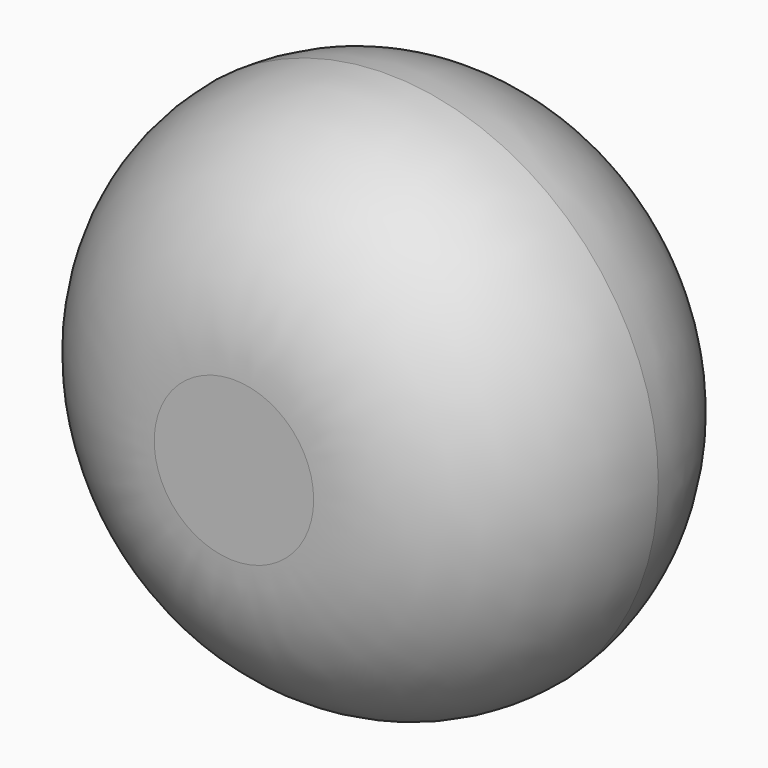
from build123d import *

# Parameters (mm, degrees)
F0_R     = 38.216457182
F1_DEPTH = 54.356
F2_R     = 26.9812507731


# Not quite as in the source:
# - a fillet or chamfer that OpenCascade refuses, or shapes differently, is made with other operations: its cross-section is extruded or revolved along the edge and cut away or added


with BuildPart() as f1:
    # F0 (on Front) → F1 (new body)
    with BuildSketch(Plane.XZ):
        with Locations((0, 37.4543480575)):
            Circle(F0_R)
    extrude(amount=F1_DEPTH)

    # F2
    f2_edges = [f1.edges().sort_by_distance(p)[0] for p in [
        (-38.216457, -54.356, 37.454348),
    ]]
    fillet(f2_edges, radius=F2_R)

    # F3: fillet of radius 29.4340917525 on 1 edges, made by hand

    # F3_s1 → F3_t2 (revolve, cut)
    with BuildSketch(Plane.XY.offset(37.4543480575)):
        with BuildLine():
            ThreePointArc((38.216457182, -27.3747492269), (28.9262515546, -7.9052664926), (8.8544942767, 0))
            Line((8.8544942767, 0), (8.8544942767, 0.588681835))
            Line((8.8544942767, 0.588681835), (38.216457182, 0.588681835))
            Line((38.216457182, 0.588681835), (38.8051390171, 0))
            ThreePointArc((38.8051390171, 0), (38.8051390171, -13.6873746135), (38.8036964401, -27.3335623764))
            Line((38.8036964401, -27.3335623764), (38.216457182, -27.3747492269))
        make_face()
    revolve(axis=Axis((0, 0, 37.4543480575), (0, -1, 0)), mode=Mode.SUBTRACT)


solid = f1.part
